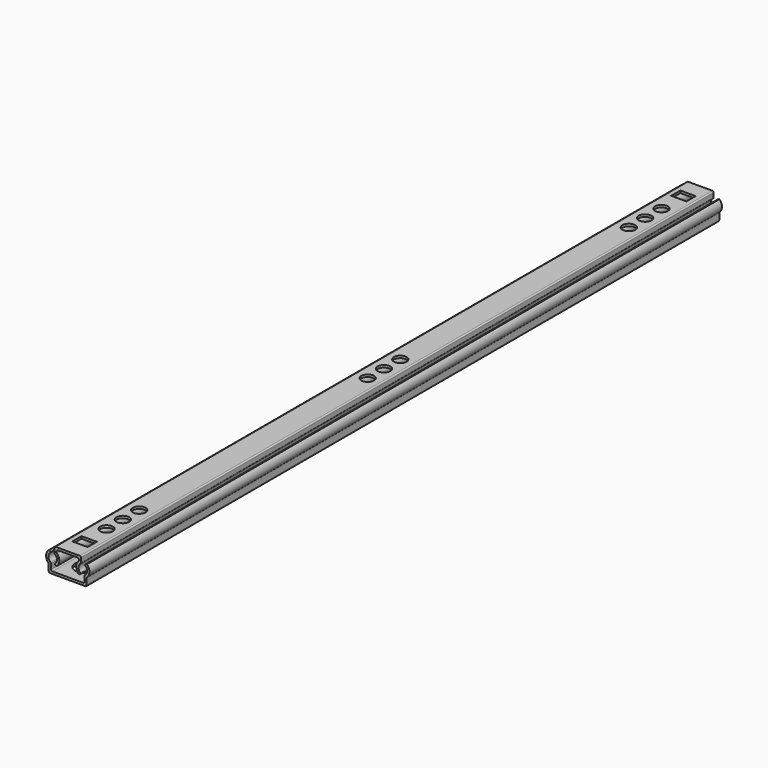
from build123d import *

# Parameters (mm, degrees)
F1_DEPTH = 310
F2_R     = 2.65
F2_R_2   = 3.9
F2_R_3   = 2
F3_DEPTH = 25
F4_DEPTH = 310
F5_R     = 2.5
F5_W     = 6
F5_H     = 4.5
F6_DEPTH = 25


with BuildPart() as f1:
    # F0 (on Front) → F1 (new body)
    with BuildSketch(Plane.XZ):
        with BuildLine():
            Line((-6.95, 0), (0, 0))
            Line((0, 0), (6.95, 0))
            ThreePointArc((6.95, 0), (7.3035533906, 0.1464466094), (7.45, 0.5))
            Line((7.45, 0.5), (7.45, 3.0193872726))
            ThreePointArc((7.45, 3.0193872726), (7.4890054933, 3.212995291), (7.5999362592, 3.3763962044))
            ThreePointArc((7.5999362592, 3.3763962044), (8.499844681, 5.5500466323), (7.5558992874, 7.70493838))
            ThreePointArc((7.5558992874, 7.70493838), (7.4469022544, 7.7573324959), (7.3276329598, 7.7373241989))
            Line((7.3276329598, 7.7373241989), (6.8485098701, 7.4919196896))
            ThreePointArc((6.8485098701, 7.4919196896), (6.7407174594, 7.3342063431), (6.8144466754, 7.1579772133))
            ThreePointArc((6.8144466754, 7.1579772133), (7.5996272621, 5.4799335442), (6.7518075872, 3.8326506577))
            ThreePointArc((6.7518075872, 3.8326506577), (6.6032919262, 3.6559163242), (6.55, 3.4313013274))
            Line((6.55, 3.4313013274), (6.55, 1.4))
            ThreePointArc((6.55, 1.4), (6.4035533906, 1.0464466094), (6.05, 0.9))
            Line((6.05, 0.9), (0, 0.9))
            Line((0, 0.9), (-6.05, 0.9))
            ThreePointArc((-6.05, 0.9), (-6.4035533906, 1.0464466094), (-6.55, 1.4))
            Line((-6.55, 1.4), (-6.55, 3.4313013274))
            ThreePointArc((-6.55, 3.4313013274), (-6.6032919262, 3.6559163242), (-6.7518075872, 3.8326506577))
            ThreePointArc((-6.7518075872, 3.8326506577), (-7.5996272621, 5.4799335442), (-6.8144466754, 7.1579772133))
            ThreePointArc((-6.8144466754, 7.1579772133), (-6.7407174594, 7.3342063431), (-6.8485098701, 7.4919196896))
            Line((-6.8485098701, 7.4919196896), (-7.3276329598, 7.7373241989))
            ThreePointArc((-7.3276329598, 7.7373241989), (-7.4469022544, 7.7573324959), (-7.5558992874, 7.70493838))
            ThreePointArc((-7.5558992874, 7.70493838), (-8.499844681, 5.5500466323), (-7.5999362592, 3.3763962044))
            ThreePointArc((-7.5999362592, 3.3763962044), (-7.4890054933, 3.212995291), (-7.45, 3.0193872726))
            Line((-7.45, 3.0193872726), (-7.45, 0.5))
            ThreePointArc((-7.45, 0.5), (-7.3035533906, 0.1464466094), (-6.95, 0))
        make_face()
    extrude(amount=F1_DEPTH)

    # F2 (on face) → F3 (cut)
    with BuildSketch(Plane(origin=(0, 0, 0), x_dir=(1, 0, 0), z_dir=(0, 0, -1))):
        with Locations((0, 10)):
            Circle(F2_R)
        with Locations((0, 301.5)):
            Circle(F2_R_2)
        with Locations((0, 278)):
            Circle(F2_R_3)
        with Locations((0, 266)):
            Circle(F2_R_3)
        with BuildLine():
            ThreePointArc((3.75, 243), (0, 246.75), (-3.75, 243))
            Line((-3.75, 243), (-3.75, 237))
            ThreePointArc((-3.75, 237), (0, 233.25), (3.75, 237))
            Line((3.75, 237), (3.75, 243))
        make_face()
        with BuildLine():
            ThreePointArc((0.9909234186, 223.1344275955), (0.6578648814, 223.7531359756), (0, 224))
            ThreePointArc((0, 224), (-0.6578648814, 223.7531359756), (-0.9909234186, 223.1344275955))
            Line((-0.9909234186, 223.1344275955), (-2.7409234186, 210.2344275955))
            ThreePointArc((-2.7409234186, 210.2344275955), (-2.5031359756, 209.4421351186), (-1.75, 209.1))
            Line((-1.75, 209.1), (0, 209.1))
            Line((0, 209.1), (1.75, 209.1))
            ThreePointArc((1.75, 209.1), (2.5031359756, 209.4421351186), (2.7409234186, 210.2344275955))
            Line((2.7409234186, 210.2344275955), (0.9909234186, 223.1344275955))
        make_face()
    extrude(amount=-F3_DEPTH, mode=Mode.SUBTRACT)


with BuildPart() as f4:
    # F0 (on Front) → F4 (new body, through all)
    with BuildSketch(Plane.XZ):
        with BuildLine():
            Line((4.75, 9.8), (0, 9.8))
            Line((0, 9.8), (-4.75, 9.8))
            ThreePointArc((-4.75, 9.8), (-5.1035533906, 9.6535533906), (-5.25, 9.3))
            Line((-5.25, 9.3), (-5.25, 7.6077230629))
            ThreePointArc((-5.25, 7.6077230629), (-5.1967080738, 7.383108066), (-5.0481924128, 7.2063737325))
            ThreePointArc((-5.0481924128, 7.2063737325), (-4.2003727379, 5.559090846), (-4.9855533246, 3.8810471769))
            ThreePointArc((-4.9855533246, 3.8810471769), (-5.0592825406, 3.7048180472), (-4.9514901299, 3.5471047007))
            Line((-4.9514901299, 3.5471047007), (-4.4723670402, 3.3017001913))
            ThreePointArc((-4.4723670402, 3.3017001913), (-4.3530977456, 3.2816918943), (-4.2441007126, 3.3340860103))
            ThreePointArc((-4.2441007126, 3.3340860103), (-3.300155319, 5.488977758), (-4.2000637408, 7.6626281859))
            ThreePointArc((-4.2000637408, 7.6626281859), (-4.3109945067, 7.8260290992), (-4.35, 8.0196371176))
            Line((-4.35, 8.0196371176), (-4.35, 8.4))
            ThreePointArc((-4.35, 8.4), (-4.2035533906, 8.7535533906), (-3.85, 8.9))
            Line((-3.85, 8.9), (0, 8.9))
            Line((0, 8.9), (3.85, 8.9))
            ThreePointArc((3.85, 8.9), (4.2035533906, 8.7535533906), (4.35, 8.4))
            Line((4.35, 8.4), (4.35, 8.0196371176))
            ThreePointArc((4.35, 8.0196371176), (4.3109945067, 7.8260290992), (4.2000637408, 7.6626281859))
            ThreePointArc((4.2000637408, 7.6626281859), (3.300155319, 5.488977758), (4.2441007126, 3.3340860103))
            ThreePointArc((4.2441007126, 3.3340860103), (4.3530977456, 3.2816918943), (4.4723670402, 3.3017001913))
            Line((4.4723670402, 3.3017001913), (4.9514901299, 3.5471047007))
            ThreePointArc((4.9514901299, 3.5471047007), (5.0592825406, 3.7048180472), (4.9855533246, 3.8810471769))
            ThreePointArc((4.9855533246, 3.8810471769), (4.2003727379, 5.559090846), (5.0481924128, 7.2063737325))
            ThreePointArc((5.0481924128, 7.2063737325), (5.1967080738, 7.383108066), (5.25, 7.6077230629))
            Line((5.25, 7.6077230629), (5.25, 9.3))
            ThreePointArc((5.25, 9.3), (5.1035533906, 9.6535533906), (4.75, 9.8))
        make_face()
    extrude(amount=F4_DEPTH)

    # F5 (on face) → F6 (cut)
    with BuildSketch(Plane.XY.offset(9.8)):
        with Locations((0, -19)):
            Circle(F5_R)
        with Locations((0, -27)):
            Circle(F5_R)
        with Locations((0, -35)):
            Circle(F5_R)
        with Locations((0, -8.25)):
            Rectangle(F5_W, F5_H)
        with Locations((0, -283)):
            Circle(F5_R)
        with Locations((0, -291)):
            Circle(F5_R)
        with Locations((0, -275)):
            Circle(F5_R)
        with Locations((0, -163)):
            Circle(F5_R)
        with Locations((0, -155)):
            Circle(F5_R)
        with Locations((0, -147)):
            Circle(F5_R)
        with Locations((0, -301.75)):
            Rectangle(F5_W, F5_H)
    extrude(amount=-F6_DEPTH, mode=Mode.SUBTRACT)


solid = Compound([f1.part, f4.part])
